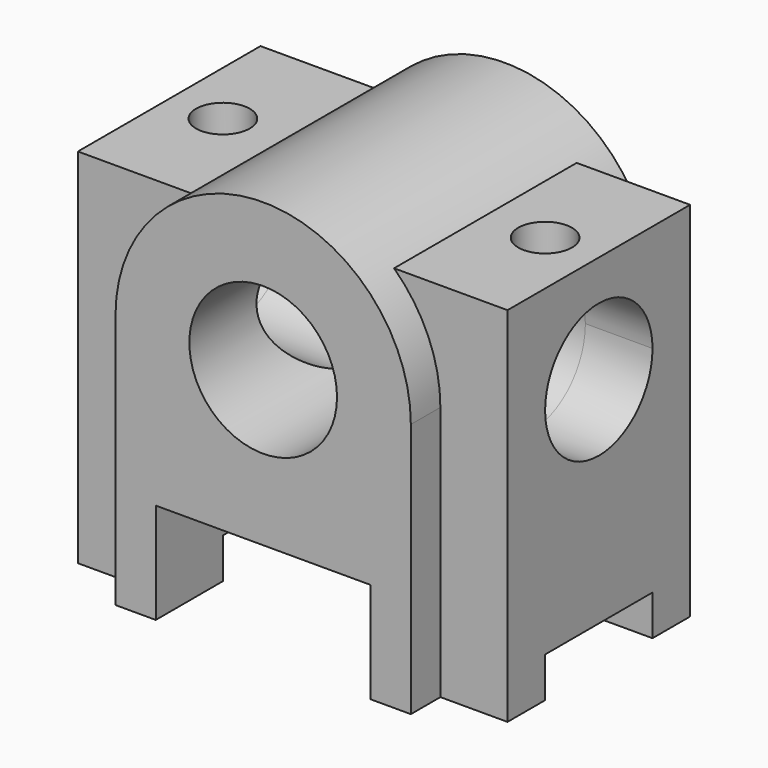
from build123d import *

# Parameters (mm, degrees)
F0_R      = 11
F0_W      = 32
F0_H      = 15
F1_DEPTH  = 22.5
F2_R      = 10
F2_W      = 20
F2_H      = 6
F3_DEPTH  = 32
F4_R      = 11
F5_DEPTH  = 45.001
F6_R      = 10
F7_DEPTH  = 64.0010001
F8_W      = 20
F8_H      = 6
F9_DEPTH  = 64.0010001
F10_W     = 32
F10_H     = 15
F11_DEPTH = 45.001
F12_R     = 4
F13_DEPTH = 15


# Not quite as in the source:
# - a pattern or mirror of a feature is missing from the dataset's text; its kind, count and spacing are read off the source's solid


with BuildPart() as f1:
    # F0 (on Front) → F1 (new body, symmetric)
    with BuildSketch(Plane.XZ):
        with BuildLine():
            Line((-22, 38), (-22, 0))
            Line((-22, 0), (-16, 0))
            Line((-16, 0), (-16, 15))
            Line((-16, 15), (16, 15))
            Line((16, 15), (16, 0))
            Line((16, 0), (22, 0))
            Line((22, 0), (22, 38))
            ThreePointArc((22, 38), (0, 60), (-22, 38))
        make_face()
        with Locations((0, 38)):
            Circle(F0_R, mode=Mode.SUBTRACT)
        with Locations((0, 7.5)):
            Rectangle(F0_W, F0_H)
    extrude(amount=F1_DEPTH, both=True)

    # F2 (on Right) → F3 (join, symmetric)
    with BuildSketch(Plane.YZ):
        Polygon((17, 0), (17, 54), (-17, 54), (-17, 0), (-10, 0), (-10, 6), (10, 6), (10, 0), align=None)
        with Locations((0, 38)):
            Circle(F2_R, mode=Mode.SUBTRACT)
        with Locations((0, 3)):
            Rectangle(F2_W, F2_H)
    extrude(amount=F3_DEPTH, both=True)

    # F4 (on face) → F5 (cut, through all)
    with BuildSketch(Plane.XZ.offset(22.5)):
        with Locations((0, 38)):
            Circle(F4_R)
    extrude(amount=-F5_DEPTH, mode=Mode.SUBTRACT)

    # F6 (on face) → F7 (cut, through all)
    with BuildSketch(Plane(origin=(-32, 0, 0), x_dir=(0, -1, 0), z_dir=(-1, 0, 0))):
        with Locations((0, 38)):
            Circle(F6_R)
    extrude(amount=-F7_DEPTH, mode=Mode.SUBTRACT)

    # F8 (on face) → F9 (cut, through all)
    with BuildSketch(Plane.YZ.offset(32)):
        with Locations((0, 3)):
            Rectangle(F8_W, F8_H)
    extrude(amount=-F9_DEPTH, mode=Mode.SUBTRACT)

    # F10 (on face) → F11 (cut, through all)
    with BuildSketch(Plane(origin=(0, 22.5, 0), x_dir=(-1, 0, 0), z_dir=(0, 1, 0))):
        with Locations((0, 7.5)):
            Rectangle(F10_W, F10_H)
    extrude(amount=-F11_DEPTH, mode=Mode.SUBTRACT)

    # F12 (on face) → F13 (cut)
    with BuildSketch(Plane.XY.offset(54)):
        with Locations((-24, 0)):
            Circle(F12_R)
    f13 = extrude(amount=-F13_DEPTH, mode=Mode.SUBTRACT)

    # F13_copies: F13 across plane
    add(f13.mirror(Plane(origin=(2.7e-05, 0, 0), x_dir=(0, 0, 1), z_dir=(1, 0, 0))), mode=Mode.SUBTRACT)


solid = f1.part
